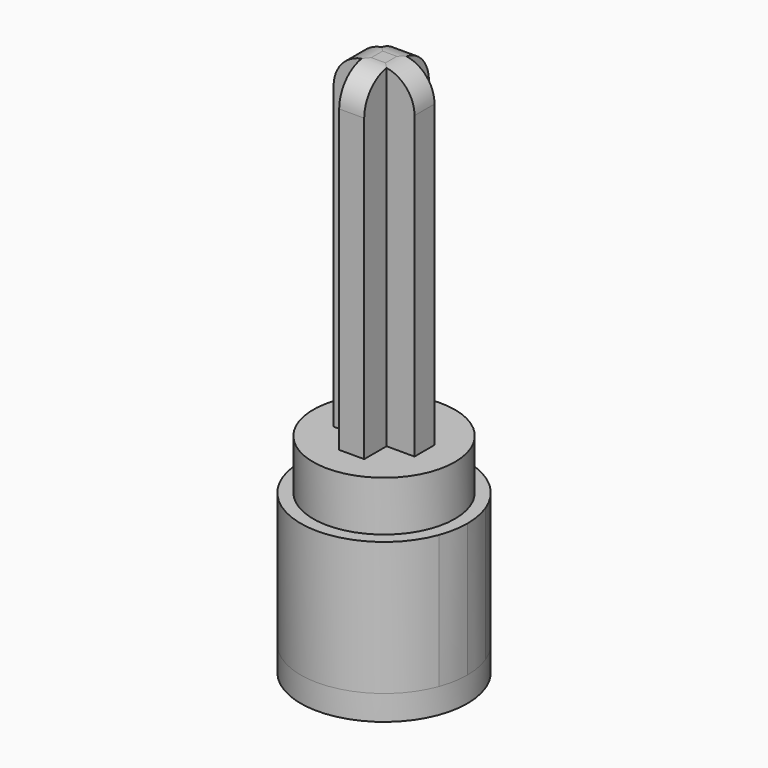
from build123d import *
from build123d import SkipClean  # not in build123d's __all__

# Parameters (mm, degrees)
F1_DEPTH    = 8
F2_R        = 4.25
F3_DEPTH    = 3
F4_W        = 1.675
F4_H        = 1.5
F4_W_2      = 1.5
F4_H_2      = 1.675
F5_DEPTH    = 20
F6_T1_DEPTH = 11.5
F6_T3_DEPTH = 11.5
F7_R        = 5
F8_DEPTH    = 1.5


# Not quite as in the source:
# - a fillet or chamfer that OpenCascade refuses, or shapes differently, is made with other operations: its cross-section is extruded or revolved along the edge and cut away or added


with BuildPart() as f1:
    # F0 (on Top) → F1 (new body)
    with BuildSketch(Plane.XY):
        with BuildLine():
            ThreePointArc((4.6837484988, -1.75), (4.9203019467, -0.8891730726), (5, 0))
            ThreePointArc((5, 0), (4.9203019467, 0.8891730726), (4.6837484988, 1.75))
            Line((4.6837484988, 1.75), (2.1213203436, 1.75))
            ThreePointArc((2.1213203436, 1.75), (2.5880621075, 0.9297497123), (2.75, 0))
            ThreePointArc((2.75, 0), (2.5880621075, -0.9297497123), (2.1213203436, -1.75))
            Line((2.1213203436, -1.75), (4.6837484988, -1.75))
        make_face()
        with BuildLine():
            Line((2.1213203436, 1.75), (4.6837484988, 1.75))
            ThreePointArc((4.6837484988, 1.75), (0, 5), (-4.6837484988, 1.75))
            Line((-4.6837484988, 1.75), (-2.1213203436, 1.75))
            ThreePointArc((-2.1213203436, 1.75), (0, 2.75), (2.1213203436, 1.75))
        make_face()
        with BuildLine():
            ThreePointArc((-4.6837484988, -1.75), (0, -5), (4.6837484988, -1.75))
            Line((4.6837484988, -1.75), (2.1213203436, -1.75))
            ThreePointArc((2.1213203436, -1.75), (0, -2.75), (-2.1213203436, -1.75))
            Line((-2.1213203436, -1.75), (-4.6837484988, -1.75))
        make_face()
        with BuildLine():
            Line((-2.1213203436, 1.75), (-4.6837484988, 1.75))
            ThreePointArc((-4.6837484988, 1.75), (-5, 0), (-4.6837484988, -1.75))
            Line((-4.6837484988, -1.75), (-2.1213203436, -1.75))
            ThreePointArc((-2.1213203436, -1.75), (-2.75, 0), (-2.1213203436, 1.75))
        make_face()
        with BuildLine():
            Line((-2.1213203436, 1.75), (2.1213203436, 1.75))
            ThreePointArc((2.1213203436, 1.75), (0, 2.75), (-2.1213203436, 1.75))
        make_face()
        with BuildLine():
            ThreePointArc((-2.1213203436, -1.75), (0, -2.75), (2.1213203436, -1.75))
            Line((2.1213203436, -1.75), (-2.1213203436, -1.75))
        make_face()
    extrude(amount=F1_DEPTH)

    # F2 (on face) → F3 (join)
    with BuildSketch(Plane.XY.offset(8)):
        Circle(F2_R)
    extrude(amount=F3_DEPTH)

    # F4 (on face) → F5 (join)
    with BuildSketch(Plane.XY.offset(11)):
        with Locations((-1.5875, 0)):
            Rectangle(F4_W, F4_H)
        Rectangle(F4_W_2, F4_H)
        with Locations((0, 1.5875)):
            Rectangle(F4_W_2, F4_H_2)
        with Locations((1.5875, 0)):
            Rectangle(F4_W, F4_H)
        with Locations((0, -1.5875)):
            Rectangle(F4_W_2, F4_H_2)
    extrude(amount=F5_DEPTH)

    # F6: fillet of radius 2 on 4 edges, made by hand

    # F6_s2 → F6_t1 (cut)
    with BuildSketch(Plane.YZ.offset(-5.75)):
        with BuildLine():
            ThreePointArc((2.425, 29), (1.8392135624, 30.4142135624), (0.425, 31))
            Line((0.425, 31), (2.425, 31))
            Line((2.425, 31), (2.425, 29))
        make_face()
        with BuildLine():
            ThreePointArc((-2.425, 29), (-1.8392135624, 30.4142135624), (-0.425, 31))
            Line((-0.425, 31), (-2.425, 31))
            Line((-2.425, 31), (-2.425, 29))
        make_face()
    extrude(amount=F6_T1_DEPTH, mode=Mode.SUBTRACT)

    # F6_s4 → F6_t3 (cut)
    with BuildSketch(Plane.XZ.offset(-5.75)):
        with BuildLine():
            ThreePointArc((2.425, 29), (1.8392135624, 30.4142135624), (0.425, 31))
            Line((0.425, 31), (2.425, 31))
            Line((2.425, 31), (2.425, 29))
        make_face()
        with BuildLine():
            ThreePointArc((-2.425, 29), (-1.8392135624, 30.4142135624), (-0.425, 31))
            Line((-0.425, 31), (-2.425, 31))
            Line((-2.425, 31), (-2.425, 29))
        make_face()
    extrude(amount=F6_T3_DEPTH, mode=Mode.SUBTRACT)

    # F7 (on face) → F8 (join)
    with BuildSketch(Plane(origin=(0, 0, 0), x_dir=(1, 0, 0), z_dir=(0, 0, -1))):
        Circle(F7_R)
        with BuildLine():
            ThreePointArc((2.1213203436, 1.75), (2.5880621075, 0.9297497123), (2.75, 0))
            ThreePointArc((2.75, 0), (2.5880621075, -0.9297497123), (2.1213203436, -1.75))
            ThreePointArc((2.1213203436, -1.75), (0, -2.75), (-2.1213203436, -1.75))
            ThreePointArc((-2.1213203436, -1.75), (-2.75, 0), (-2.1213203436, 1.75))
            ThreePointArc((-2.1213203436, 1.75), (0, 2.75), (2.1213203436, 1.75))
        make_face(mode=Mode.SUBTRACT)
    with SkipClean():  # cleaning this boolean's faces spoils the solid; the shape is the same uncleaned
        extrude(amount=F8_DEPTH)


solid = f1.part
